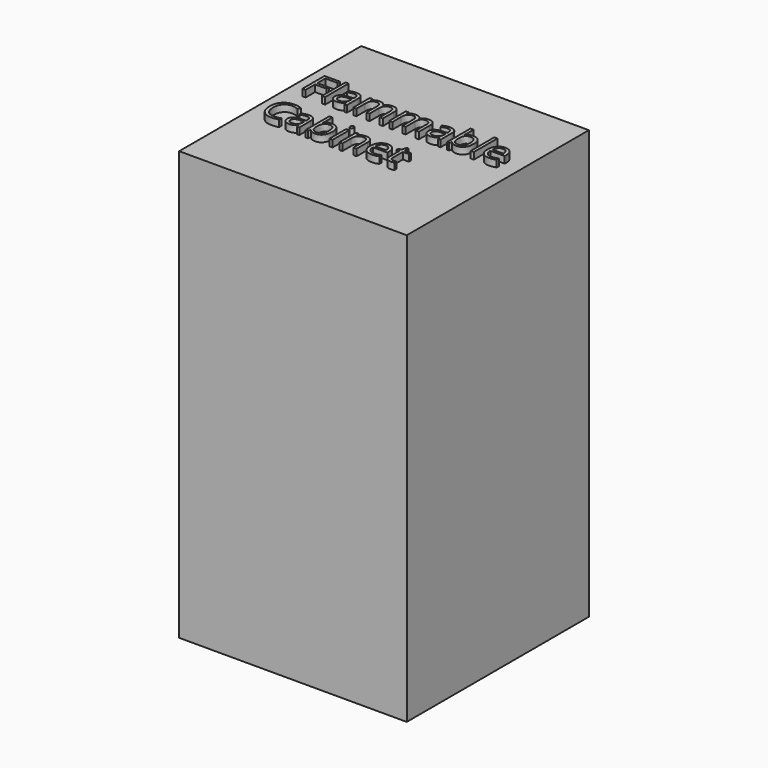
from build123d import *

# Parameters (mm, degrees)
F0_W         = 863.6
F0_H         = 863.6
F1_DEPTH     = 1625.6
F2_TEXT_SIZE = 147.077628325
F3_DEPTH     = 25.4


# Not quite as in the source:
# - Text() gives the source's letters only with a copy of the font that has no kerning and outlines rounded to 1/6400 em; it was checked with that copy


with BuildPart() as f1:
    # F0 (on Top) → F1 (new body)
    with BuildSketch(Plane.XY):
        Rectangle(F0_W, F0_H)
    extrude(amount=F1_DEPTH)

    # F2 (on face) → F3 (join)
    with BuildSketch(Plane.XY.offset(1625.6)):
        with Locations((-381, 70.9813116716)):
            Text('Flammable', F2_TEXT_SIZE, font='Open Sans', text_align=(TextAlign.LEFT, TextAlign.BOTTOM))
        with Locations((-381, -129.0442628504)):
            Text('Cabinet', F2_TEXT_SIZE, font='Open Sans', text_align=(TextAlign.LEFT, TextAlign.BOTTOM))
    extrude(amount=F3_DEPTH)


solid = f1.part
